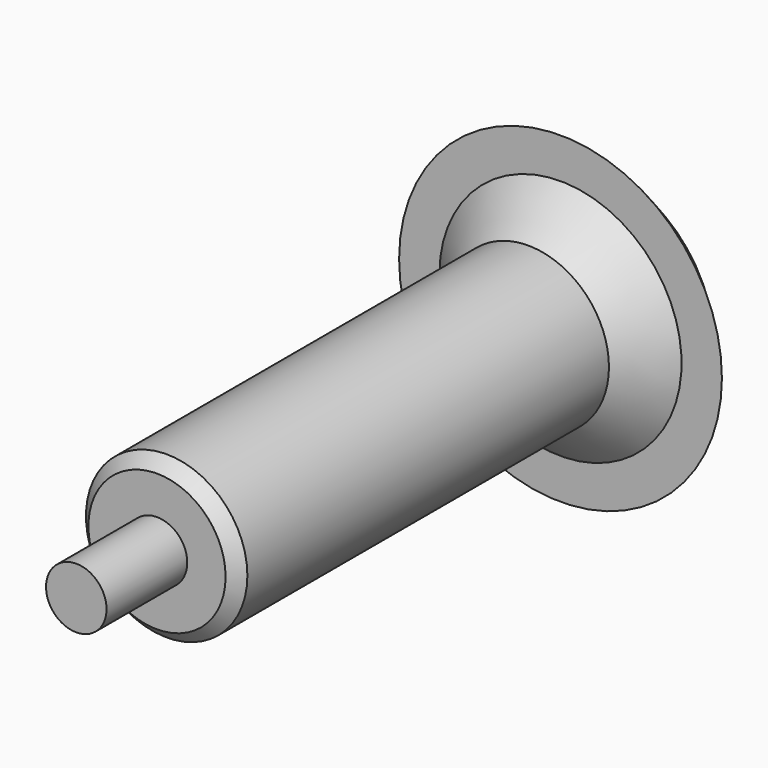
from build123d import *

# Parameters (mm, degrees)
F0_R     = 20
F1_DEPTH = 115
F2_SIZE  = 3
F3_R     = 7.5
F4_DEPTH = 25
F5_R     = 30
F6_DEPTH = 10
F7_R     = 40
F8_DEPTH = 10
F9_SIZE  = 9.99999


# Not quite as in the source:
# - a fillet or chamfer is up to 0.001 mm smaller than in the source, because OpenCascade refuses the exact size


with BuildPart() as f1:
    # F0 (on Front) → F1 (new body)
    with BuildSketch(Plane.XZ):
        Circle(F0_R)
    extrude(amount=F1_DEPTH)

    # F2
    f2_edges = [f1.edges().sort_by_distance(p)[0] for p in [
        (-20, -115, 0),
    ]]
    chamfer(f2_edges, length=F2_SIZE)

    # F3 (on face) → F4 (join)
    with BuildSketch(Plane.XZ.offset(115)):
        Circle(F3_R)
    extrude(amount=F4_DEPTH)

    # F5 (on face) → F6 (join)
    with BuildSketch(Plane(origin=(0, 0, 0), x_dir=(-1, 0, 0), z_dir=(0, 1, 0))):
        Circle(F5_R)
    extrude(amount=F6_DEPTH)

    # F7 (on face) → F8 (join)
    with BuildSketch(Plane(origin=(0, 10, 0), x_dir=(-1, 0, 0), z_dir=(0, 1, 0))):
        Circle(F7_R)
    extrude(amount=F8_DEPTH)

    # F9 (size 10 in the source; OpenCascade refuses exactly that, so slightly less here)
    f9_edges = [f1.edges().sort_by_distance(p)[0] for p in [
        (40, 20, 0),
        (30, 0, 0),
    ]]
    chamfer(f9_edges, length=F9_SIZE)


solid = f1.part
